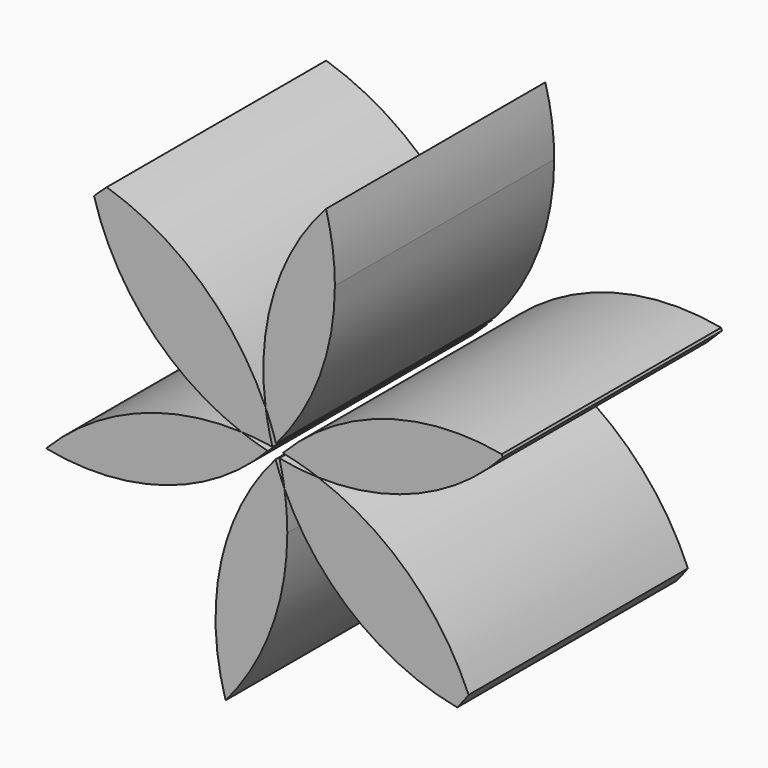
from build123d import *

# Parameters (mm, degrees)
F1_DEPTH = 25.4


with BuildPart() as f1:
    # F0 (on Front) → F1 (new body)
    with BuildSketch(Plane.XZ):
        with BuildLine():
            ThreePointArc((4.6213866978, -0.0897776155), (13.9343103429, 1.6461109528), (21.6857667516, 7.0920984194))
            ThreePointArc((21.6857667516, 7.0920984194), (21.6461431831, 7.2121303992), (21.6058552362, 7.3319410193))
            ThreePointArc((21.6058552362, 7.3319410193), (10.6469893917, 6.6485268007), (1.3317239543, 0.8356423686))
            ThreePointArc((1.3317239543, 0.8356423686), (2.9931346457, 0.4318681801), (4.6213866978, -0.0897776155))
        make_face()
    extrude(amount=F1_DEPTH)


with BuildPart() as f1b:
    # F0 (on Front) → F1, piece 2 (new body)
    with BuildSketch(Plane.XZ):
        with BuildLine():
            ThreePointArc((17.4770130194, -14.6671181736), (18.0203473677, -13.9941923791), (18.5377871083, -13.3011574205))
            ThreePointArc((18.5377871083, -13.3011574205), (12.9653166545, -5.2357887889), (4.6213866978, -0.0897776155))
            ThreePointArc((4.6213866978, -0.0897776155), (2.8062647028, 0.0386290803), (1.007659838, 0.3146303056))
            ThreePointArc((1.007659838, 0.3146303056), (1.2704089268, -0.8386508434), (1.4757043874, -2.0035320674))
            ThreePointArc((1.4757043874, -2.0035320674), (7.9321763784, -10.2865052807), (17.4770130194, -14.6671181736))
        make_face()
    extrude(amount=F1_DEPTH)


with BuildPart() as f1c:
    # F0 (on Front) → F1, piece 3 (new body)
    with BuildSketch(Plane.XZ):
        with BuildLine():
            ThreePointArc((1.7425521853, -5.5627638467), (1.6757467511, -3.7781533426), (1.4757043874, -2.0035320674))
            ThreePointArc((1.4757043874, -2.0035320674), (1.0387881275, -0.9626758426), (0.6554370266, 0.0990771571))
            ThreePointArc((0.6554370266, 0.0990771571), (-4.3891058934, -9.8839406609), (-3.9733789111, -21.0613835304))
            ThreePointArc((-3.9733789111, -21.0613835304), (0.2680264287, -13.8222898682), (1.7425521853, -5.5627638467))
        make_face()
    extrude(amount=F1_DEPTH)


with BuildPart() as f1d:
    # F0 (on Front) → F1, piece 4 (new body)
    with BuildSketch(Plane.XZ):
        with BuildLine():
            ThreePointArc((6.1509268163, 16.032225236), (5.9442716589, 19.0668842682), (5.3281218462, 22.0455116708))
            ThreePointArc((5.3281218462, 22.0455116708), (0.5167522435, 13.6533436879), (-0.261552872, 4.011144662))
            ThreePointArc((-0.261552872, 4.011144662), (0.2598824531, 2.7188109382), (0.7050131891, 1.3982504966))
            ThreePointArc((0.7050131891, 1.3982504966), (4.7453171219, 8.2249979448), (6.1509268163, 16.032225236))
        make_face()
    extrude(amount=F1_DEPTH)


with BuildPart() as f1e:
    # F0 (on Front) → F1, piece 5 (new body)
    with BuildSketch(Plane.XZ):
        with BuildLine():
            ThreePointArc((-0.261552872, 4.011144662), (-6.1889624772, 12.2063757044), (-14.977916047, 17.2114023393))
            ThreePointArc((-14.977916047, 17.2114023393), (-15.5794327412, 16.6688816379), (-16.1613123945, 16.1053507036))
            ThreePointArc((-16.1613123945, 16.1053507036), (-11.0976151814, 7.074124231), (-2.5004444077, 1.3041384638))
            ThreePointArc((-2.5004444077, 1.3041384638), (-1.0633867227, 1.2021041869), (0.3649000763, 1.0135767259))
            ThreePointArc((0.3649000763, 1.0135767259), (0.3680275088, 1.0170339184), (0.3711542213, 1.020491762))
            ThreePointArc((0.3711542213, 1.020491762), (0.0031770858, 2.5048966467), (-0.261552872, 4.011144662))
        make_face()
    extrude(amount=F1_DEPTH)


with BuildPart() as f1f:
    # F0 (on Front) → F1, piece 6 (new body)
    with BuildSketch(Plane.XZ):
        with BuildLine():
            ThreePointArc((-20.6031874455, -5.9219877035), (-9.5043648842, -5.3170713225), (-0.0648176749, 0.5518923477))
            ThreePointArc((-0.0648176749, 0.5518923477), (-1.2933910681, 0.8931765303), (-2.5004444077, 1.3041384638))
            ThreePointArc((-2.5004444077, 1.3041384638), (-12.3228568037, -0.3773288316), (-20.6031874455, -5.9219877035))
        make_face()
    extrude(amount=F1_DEPTH)


solid = Compound([f1.part, f1b.part, f1c.part, f1d.part, f1e.part, f1f.part])
